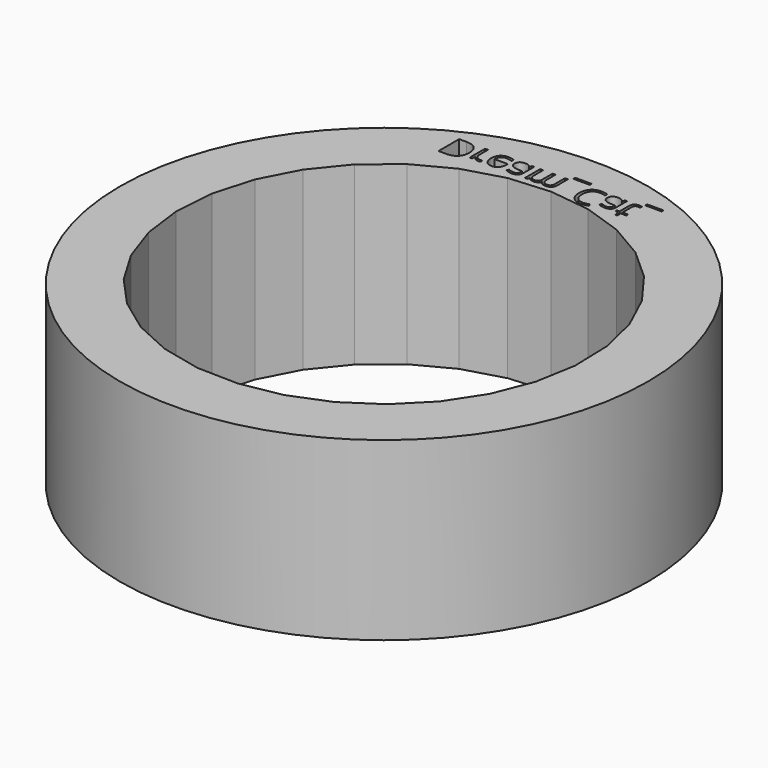
from build123d import *

# Parameters (mm, degrees)
F0_R         = 76.1423222344
F1_DEPTH     = 25.4
F2_TEXT_SIZE = 10.428923027
F3_DEPTH     = 25.4
F4_DEPTH     = 25.4
F6_DEPTH     = 25.4
F7_DEPTH     = 25.4


# Not quite as in the source:
# - Text() gives the source's letters only with a copy of the font that has no kerning and outlines rounded to 1/6400 em; it was checked with that copy


with BuildPart() as f1:
    # F0 (on Top) → F1 (new body)
    with BuildSketch(Plane.XY):
        Circle(F0_R)
    extrude(amount=F1_DEPTH)

    # F2 (on face) → F3 (cut)
    with BuildSketch(Plane(origin=(0, 0, 0), x_dir=(1, 0, 0), z_dir=(0, 0, -1))):
        with Locations((-31.9125011592, -65.6922003254)):
            Text('Dream_Cat_', F2_TEXT_SIZE, font='Open Sans', text_align=(TextAlign.LEFT, TextAlign.BOTTOM))
    extrude(amount=-F3_DEPTH, mode=Mode.SUBTRACT)

    # F4 (add): a face of the model
    f4_faces = [f1.faces().sort_by_distance(p)[0] for p in [
        (0.0625524275, -0.482402401, 25.4),
    ]]
    extrude(f4_faces, amount=F4_DEPTH)

    # F5 (on face) → F6 (cut)
    with BuildSketch(Plane(origin=(0, 0, 0), x_dir=(1, 0, 0), z_dir=(0, 0, -1))):
        Polygon((24.3243419531, -53.3579662511), (34.5673008856, -47.36927151), (43.3950704584, -39.4412732276), (50.4462407479, -29.8985445851), (55.432136014, -19.1317660144), (58.1486331186, -7.5817306952), (58.4845183513, 4.2787015695), (56.426040531, 15.9639632892), (52.0574739815, 26.9956584762), (45.5576683308, 36.9221482333), (37.1927263858, 45.3370409035), (27.3051098526, 51.8958297923), (16.2996189139, 56.3299973119), (4.6268196617, 58.4580081231), (-7.2354021311, 58.1927412132), (-18.8014057106, 55.5450566406), (-29.5976775311, 50.6233509229), (-39.182216956, 43.6291192705), (-47.1626318149, 34.8487063489), (-53.212202986, 24.6415832948), (-57.0832603147, 13.4256309254), (-58.6173222591, 1.6600316484), (-57.751584143, -10.1735295193), (-54.5214893865, -21.5905851931), (-49.0592784485, -32.1237197723), (-41.5885748867, -41.3417054897), (-32.4152301825, -48.8671569269), (-21.914802146, -54.3919812178), (-10.5171795348, -57.6899914069), (1.3110176423, -58.6261665696), (13.0855416031, -57.1621795845), align=None)
    extrude(amount=-F6_DEPTH, mode=Mode.SUBTRACT)

    # F7 (cut): a face of the model
    f7_faces = [f1.faces().sort_by_distance(p)[0] for p in [
        (0, 0, 25.4),
    ]]
    extrude(f7_faces, amount=-F7_DEPTH, mode=Mode.SUBTRACT)


solid = f1.part
